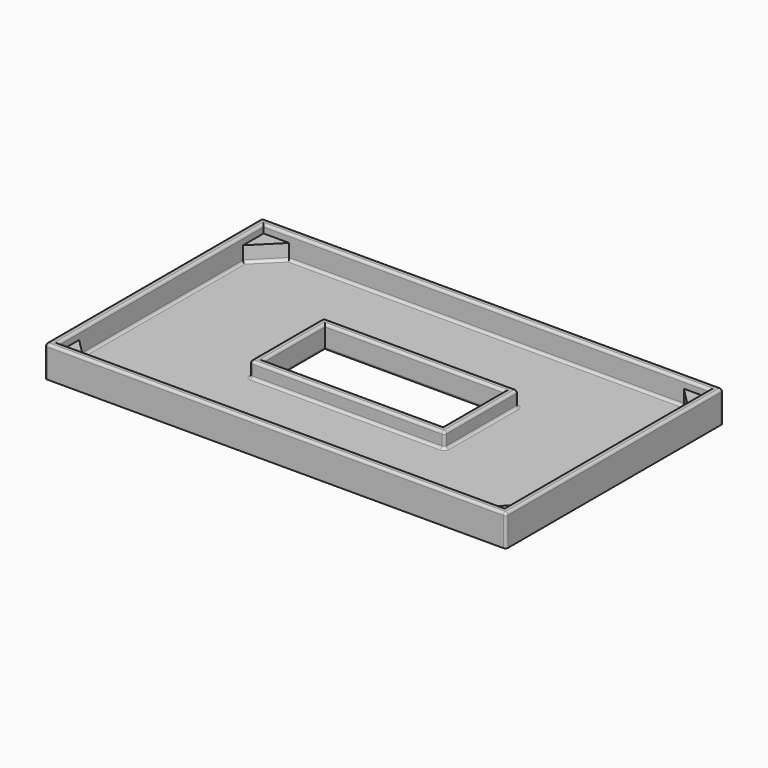
from build123d import *

# Parameters (mm, degrees)
F1_W     = 90
F1_H     = 53
F1_W_2   = 35
F1_H_2   = 15
F2_DEPTH = 1.5
F3_W     = 90
F3_H     = 53
F3_W_2   = 87
F3_H_2   = 50
F4_DEPTH = 4.6
F5_W     = 38
F5_H     = 18
F5_W_2   = 35
F5_H_2   = 15
F6_DEPTH = 3
F7_R     = 0.5


with BuildPart() as f2:
    # F1 (on Top) → F2 (new body)
    with BuildSketch(Plane.XY):
        Rectangle(F1_W, F1_H)
        Rectangle(F1_W_2, F1_H_2, mode=Mode.SUBTRACT)
    extrude(amount=F2_DEPTH)

    # F3 (on face) → F4 (join)
    with BuildSketch(Plane.XY.offset(1.5)):
        Rectangle(F3_W, F3_H)
        Rectangle(F3_W_2, F3_H_2, mode=Mode.SUBTRACT)
    extrude(amount=F4_DEPTH)

    # F5 (on face) → F6 (join)
    with BuildSketch(Plane.XY.offset(1.5)):
        Polygon((-38.5, 25), (-43.5, 25), (-43.5, 20), align=None)
        Polygon((43.5, 20), (43.5, 25), (38.5, 25), align=None)
        Polygon((-43.5, -20), (-43.5, -25), (-38.5, -25), align=None)
        Polygon((38.5, -25), (43.5, -25), (43.5, -20), align=None)
        Rectangle(F5_W, F5_H)
        Rectangle(F5_W_2, F5_H_2, mode=Mode.SUBTRACT)
    extrude(amount=F6_DEPTH)

    # F7
    f7_edges = [f2.edges().sort_by_distance(p)[0] for p in [
        (-45, -26.5, 3.05),
        (45, -26.5, 3.05),
        (45, 26.5, 3.05),
        (-45, 26.5, 3.05),
        (0, 26.5, 6.1),
        (-45, 0, 6.1),
        (45, 0, 6.1),
        (0, -26.5, 6.1),
        (-43.5, 0, 6.1),
        (0, 25, 6.1),
        (43.5, 0, 6.1),
        (0, -25, 6.1),
        (0, -9, 4.5),
        (19, 0, 4.5),
        (0, 7.5, 4.5),
        (0, 9, 4.5),
        (17.5, 0, 4.5),
        (-17.5, 0, 4.5),
        (-19, 0, 4.5),
        (0, 7.5, 0),
        (-17.5, 0, 0),
        (0, -7.5, 0),
        (17.5, 0, 0),
        (-19, -9, 3),
        (-19, 9, 3),
        (-19, 0, 1.5),
        (0, -7.5, 4.5),
        (19, 0, 1.5),
        (19, 9, 3),
        (19, -9, 3),
        (-43.5, 0, 1.5),
        (-41, -22.5, 1.5),
        (-41, 22.5, 1.5),
        (0, 25, 1.5),
        (41, 22.5, 1.5),
        (43.5, 0, 1.5),
        (41, -22.5, 1.5),
        (0, -25, 1.5),
        (0, 9, 1.5),
        (0, -9, 1.5),
    ]]
    fillet(f7_edges, radius=F7_R)


solid = f2.part
